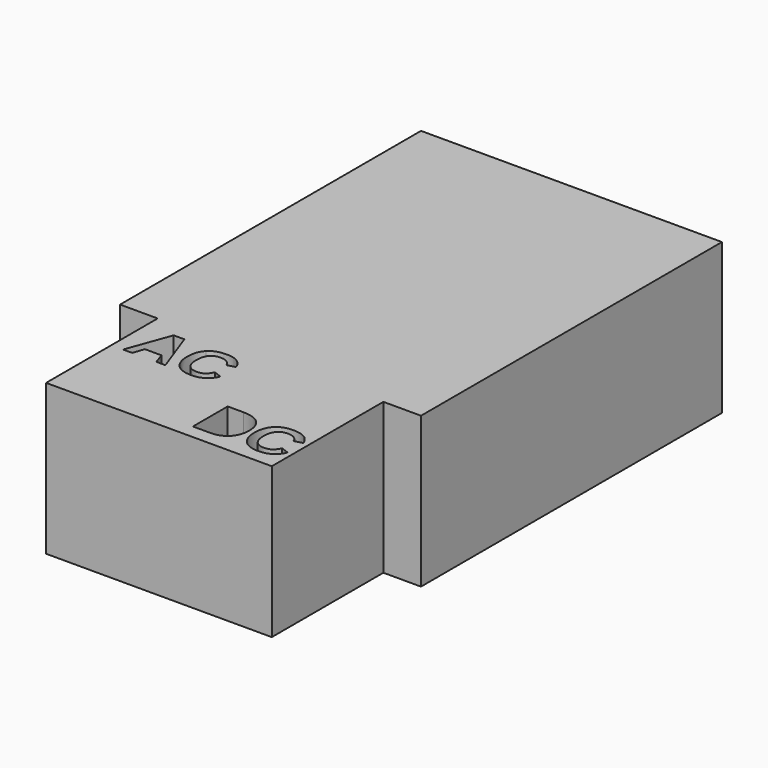
from build123d import *

# Parameters (mm, degrees)
F1_DEPTH = 203.2


with BuildPart() as f1:
    # F0 (on Top) → F1 (new body)
    with BuildSketch(Plane.XY):
        Polygon((214.0153056353, 225.6372907119), (-192.3846943647, 225.6372907119), (-192.3846943647, -282.3627092881), (-141.5846943647, -282.3627092881), (163.2153056353, -282.3627092881), (214.0153056353, -282.3627092881), align=None)
        Polygon((163.2153056353, -282.3627092881), (-141.5846943647, -282.3627092881), (-141.5846943647, -470.7070589066), align=None)
        Polygon((-68.5457757791, -360.5891466141), (-80.6984541123, -360.5891466141), (-85.9086484415, -345.5981782754), (-108.2685105503, -345.5981782754), (-113.4787048795, -360.5891466141), (-125.7646362646, -360.5891466141), (-104.3508708244, -301.9178278628), (-89.866264083, -301.9178278628), align=None, mode=Mode.SUBTRACT)
        with BuildLine():
            add(Edge.make_bspline(
                [(-45.9926967451, -346.4243471972), (-41.5620327694, -351.7544692731), (-33.1937411102, -351.7544692731)],
                knots=[0, 0, 0, 1, 1, 1], degree=2))
            add(Edge.make_bspline(
                [(-33.1937411102, -351.7544692731), (-22.0671112766, -351.7544692731), (-17.7363870898, -340.6011888292)],
                knots=[0, 0, 0, 1, 1, 1], degree=2))
            Line((-17.7363870898, -340.6011888292), (-7.0361670223, -344.6387563017))
            add(Edge.make_bspline(
                [(-7.0361670223, -344.6387563017), (-10.4874210665, -353.1403010129), (-17.1767242718, -357.284470927)],
                knots=[0, 0, 0, 1, 1, 1], degree=2))
            add(Edge.make_bspline(
                [(-17.1767242718, -357.284470927), (-23.8660274772, -361.428640841), (-33.1937411102, -361.428640841)],
                knots=[0, 0, 0, 1, 1, 1], degree=2))
            add(Edge.make_bspline(
                [(-33.1937411102, -361.428640841), (-47.3452152219, -361.428640841), (-55.0672295794, -353.4068071167)],
                knots=[0, 0, 0, 1, 1, 1], degree=2))
            add(Edge.make_bspline(
                [(-55.0672295794, -353.4068071167), (-62.789243937, -345.3849733924), (-62.789243937, -330.980318482)],
                knots=[0, 0, 0, 1, 1, 1], degree=2))
            add(Edge.make_bspline(
                [(-62.789243937, -330.980318482), (-62.789243937, -316.5356876561), (-55.3403983358, -308.7870226882)],
                knots=[0, 0, 0, 1, 1, 1], degree=2))
            add(Edge.make_bspline(
                [(-55.3403983358, -308.7870226882), (-47.8915527347, -301.0383577202), (-33.7267533178, -301.0383577202)],
                knots=[0, 0, 0, 1, 1, 1], degree=2))
            add(Edge.make_bspline(
                [(-33.7267533178, -301.0383577202), (-23.3996417955, -301.0383577202), (-16.9035555155, -305.1825276343)],
                knots=[0, 0, 0, 1, 1, 1], degree=2))
            add(Edge.make_bspline(
                [(-16.9035555155, -305.1825276343), (-10.4074692354, -309.3266975484), (-7.7823841129, -317.3618565779)],
                knots=[0, 0, 0, 1, 1, 1], degree=2))
            Line((-7.7823841129, -317.3618565779), (-18.6158572324, -320.3200743301))
            add(Edge.make_bspline(
                [(-18.6158572324, -320.3200743301), (-19.9883636669, -315.9093983122), (-24.0059431817, -313.3043011476)],
                knots=[0, 0, 0, 1, 1, 1], degree=2))
            add(Edge.make_bspline(
                [(-24.0059431817, -313.3043011476), (-28.0235226965, -310.6992039829), (-33.4735725191, -310.6992039829)],
                knots=[0, 0, 0, 1, 1, 1], degree=2))
            add(Edge.make_bspline(
                [(-33.4735725191, -310.6992039829), (-41.8018882629, -310.6992039829), (-46.1126244918, -315.862759744)],
                knots=[0, 0, 0, 1, 1, 1], degree=2))
            add(Edge.make_bspline(
                [(-46.1126244918, -315.862759744), (-50.4233607207, -321.0263155052), (-50.4233607207, -330.980318482)],
                knots=[0, 0, 0, 1, 1, 1], degree=2))
            add(Edge.make_bspline(
                [(-50.4233607207, -330.980318482), (-50.4233607207, -341.0942251212), (-45.9926967451, -346.4243471972)],
                knots=[0, 0, 0, 1, 1, 1], degree=2))
        make_face(mode=Mode.SUBTRACT)
        Polygon((163.2153056353, -470.7070589066), (163.2153056353, -282.3627092881), (-141.5846943647, -470.7070589066), align=None)
        with BuildLine():
            add(Edge.make_bspline(
                [(85.7413243761, -400.5675143045), (93.8631018313, -408.0430141443), (93.8631018313, -421.9946154497)],
                knots=[0, 0, 0, 1, 1, 1], degree=2))
            add(Edge.make_bspline(
                [(93.8631018313, -421.9946154497), (93.8631018313, -431.0691526884), (90.3052436188, -437.8317483546)],
                knots=[0, 0, 0, 1, 1, 1], degree=2))
            add(Edge.make_bspline(
                [(90.3052436188, -437.8317483546), (86.7473854062, -444.5943440207), (80.2313080058, -448.1788528566)],
                knots=[0, 0, 0, 1, 1, 1], degree=2))
            add(Edge.make_bspline(
                [(80.2313080058, -448.1788528566), (73.7152306053, -451.7633616924), (65.2936336377, -451.7633616924)],
                knots=[0, 0, 0, 1, 1, 1], degree=2))
            Line((65.2936336377, -451.7633616924), (41.5612535758, -451.7633616924))
            Line((41.5612535758, -451.7633616924), (41.5612535758, -393.0920144647))
            Line((41.5612535758, -393.0920144647), (62.8018003578, -393.0920144647))
            add(Edge.make_bspline(
                [(62.8018003578, -393.0920144647), (77.6195469209, -393.0920144647), (85.7413243761, -400.5675143045)],
                knots=[0, 0, 0, 1, 1, 1], degree=2))
        make_face(mode=Mode.SUBTRACT)
        with BuildLine():
            add(Edge.make_bspline(
                [(117.7487229773, -437.5985554006), (122.1793891034, -442.9286800635), (130.5476848243, -442.9286800635)],
                knots=[0, 0, 0, 1, 1, 1], degree=2))
            add(Edge.make_bspline(
                [(130.5476848243, -442.9286800635), (141.6743200583, -442.9286800635), (146.0050463469, -431.7753942062)],
                knots=[0, 0, 0, 1, 1, 1], degree=2))
            Line((146.0050463469, -431.7753942062), (156.7052716079, -435.8129636385))
            add(Edge.make_bspline(
                [(156.7052716079, -435.8129636385), (153.2540158886, -444.3145124759), (146.5647094366, -448.4586844014)],
                knots=[0, 0, 0, 1, 1, 1], degree=2))
            add(Edge.make_bspline(
                [(146.5647094366, -448.4586844014), (139.8754029845, -452.6028563268), (130.5476848243, -452.6028563268)],
                knots=[0, 0, 0, 1, 1, 1], degree=2))
            add(Edge.make_bspline(
                [(130.5476848243, -452.6028563268), (116.3962038441, -452.6028563268), (108.6741857386, -444.5810187091)],
                knots=[0, 0, 0, 1, 1, 1], degree=2))
            add(Edge.make_bspline(
                [(108.6741857386, -444.5810187091), (100.9521676331, -436.5591810913), (100.9521676331, -422.1545191896)],
                knots=[0, 0, 0, 1, 1, 1], degree=2))
            add(Edge.make_bspline(
                [(100.9521676331, -422.1545191896), (100.9521676331, -407.7098813529), (108.4010168496, -399.9612126241)],
                knots=[0, 0, 0, 1, 1, 1], degree=2))
            add(Edge.make_bspline(
                [(108.4010168496, -399.9612126241), (115.8498660661, -392.2125438953), (130.014672358, -392.2125438953)],
                knots=[0, 0, 0, 1, 1, 1], degree=2))
            add(Edge.make_bspline(
                [(130.014672358, -392.2125438953), (140.3417888925, -392.2125438953), (146.8378783255, -396.3567158207)],
                knots=[0, 0, 0, 1, 1, 1], degree=2))
            add(Edge.make_bspline(
                [(146.8378783255, -396.3567158207), (153.3339677585, -400.5008877462), (155.9590541551, -408.5360506756)],
                knots=[0, 0, 0, 1, 1, 1], degree=2))
            Line((155.9590541551, -408.5360506756), (145.1255757776, -411.4942698636))
            add(Edge.make_bspline(
                [(145.1255757776, -411.4942698636), (143.7530686768, -407.083591705), (139.7354872121, -404.4784932759)],
                knots=[0, 0, 0, 1, 1, 1], degree=2))
            add(Edge.make_bspline(
                [(139.7354872121, -404.4784932759), (135.7179057474, -401.8733948469), (130.2678532795, -401.8733948469)],
                knots=[0, 0, 0, 1, 1, 1], degree=2))
            add(Edge.make_bspline(
                [(130.2678532795, -401.8733948469), (121.9395334936, -401.8733948469), (117.6287951724, -407.0369531142)],
                knots=[0, 0, 0, 1, 1, 1], degree=2))
            add(Edge.make_bspline(
                [(117.6287951724, -407.0369531142), (113.3180568512, -412.2005113814), (113.3180568512, -422.1545191896)],
                knots=[0, 0, 0, 1, 1, 1], degree=2))
            add(Edge.make_bspline(
                [(113.3180568512, -422.1545191896), (113.3180568512, -432.2684307376), (117.7487229773, -437.5985554006)],
                knots=[0, 0, 0, 1, 1, 1], degree=2))
        make_face(mode=Mode.SUBTRACT)
    extrude(amount=F1_DEPTH)


solid = f1.part
